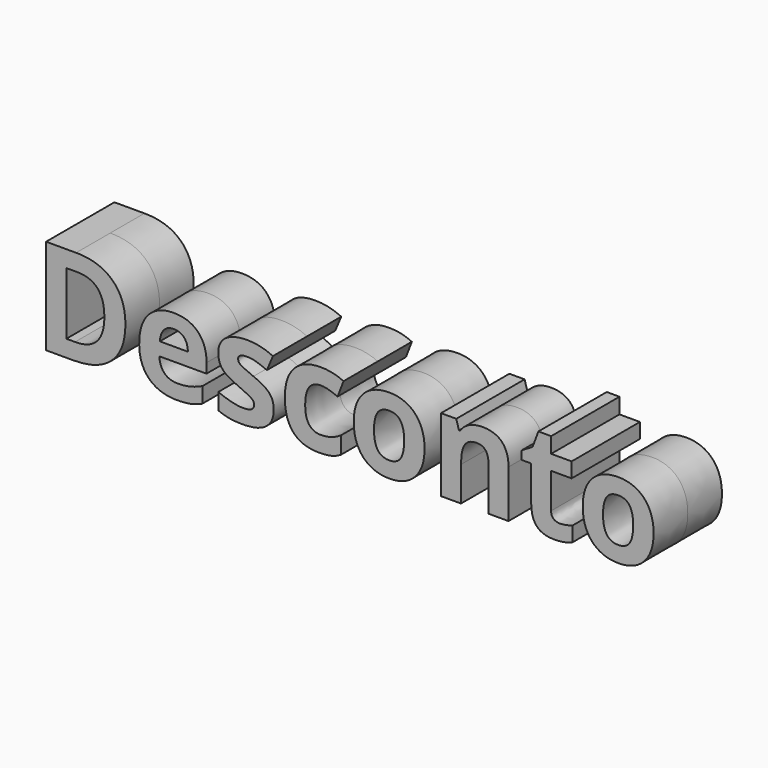
from build123d import *

# Parameters (mm, degrees)
F0_TEXT_SIZE = 78.3911181821
F1_DEPTH     = 25


# Not quite as in the source:
# - Text() gives the source's letters only with a copy of the font that has no kerning and outlines rounded to 1/6400 em; it was checked with that copy


with BuildPart() as f1:
    # F0 (on Front) → F1 (new body, symmetric)
    with BuildSketch(Plane.XZ):
        with Locations((-157.8823029995, -33.6610674858)):
            Text('Desconto', F0_TEXT_SIZE, font='Open Sans', font_style=FontStyle.BOLD, text_align=(TextAlign.LEFT, TextAlign.BOTTOM))
    extrude(amount=F1_DEPTH, both=True)


solid = f1.part
